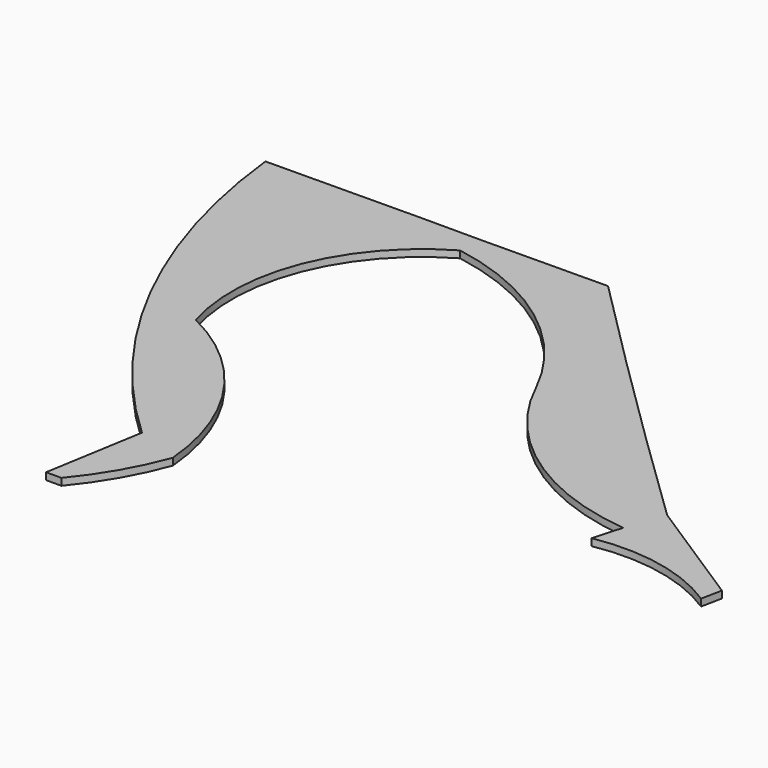
from build123d import *

# Parameters (mm, degrees)
F1_DEPTH = 2


# Not quite as in the source:
# - a feature names something its author has since deleted; it is built from what else it names


with BuildPart() as f1:
    # F0 (on Top) → F1 (new body)
    with BuildSketch(Plane.XY):
        with BuildLine():
            Line((-17.7180729806, 0), (-13.3472634479, 0))
            ThreePointArc((-13.3472634479, 0), (-5.6771986993, 10.9915241569), (0, 23.1328960508))
            ThreePointArc((0, 23.1328960508), (-11.5247073045, 55.6975197064), (-37.5854000449, 78.3715993166))
            ThreePointArc((-37.5854000449, 78.3715993166), (-36.1278357664, 114.3054992712), (-12.5523087913, 141.4636322597))
            ThreePointArc((-12.5523087913, 141.4636322597), (19.6930692126, 127.5307837734), (42.0421807398, 100.4308597236))
            ThreePointArc((42.0421807398, 100.4308597236), (65.4226402571, 72.3273330377), (99.6574273635, 59.5041723042))
            Line((99.6574273635, 59.5041723042), (97.2733384301, 51.1598982899))
            ThreePointArc((97.2733384301, 51.1598982899), (116.6670679291, 50.9395271005), (134.6239036251, 43.610314378))
            Line((134.6239036251, 43.610314378), (135.8159518172, 49.5705106347))
            Line((135.8159518172, 49.5705106347), (103.4726053476, 70.4246684909))
            ThreePointArc((103.4726053476, 70.4246684909), (63.5065429383, 109.2866549818), (24.0146897469, 148.6304431832))
            Line((24.0146897469, 148.6304431832), (-12.1552264318, 148.3045816422))
            Line((-12.1552264318, 148.3045816422), (-29.2411223054, 148.3045816422))
            Line((-29.2411223054, 148.3045816422), (-73.3465850353, 147.9072272778))
            ThreePointArc((-73.3465850353, 147.9072272778), (-53.9798913788, 82.6367857077), (-12.9499193281, 28.30594033))
            Line((-12.9499193281, 28.30594033), (-17.7180729806, 0))
        make_face()
    extrude(amount=F1_DEPTH)


solid = f1.part
